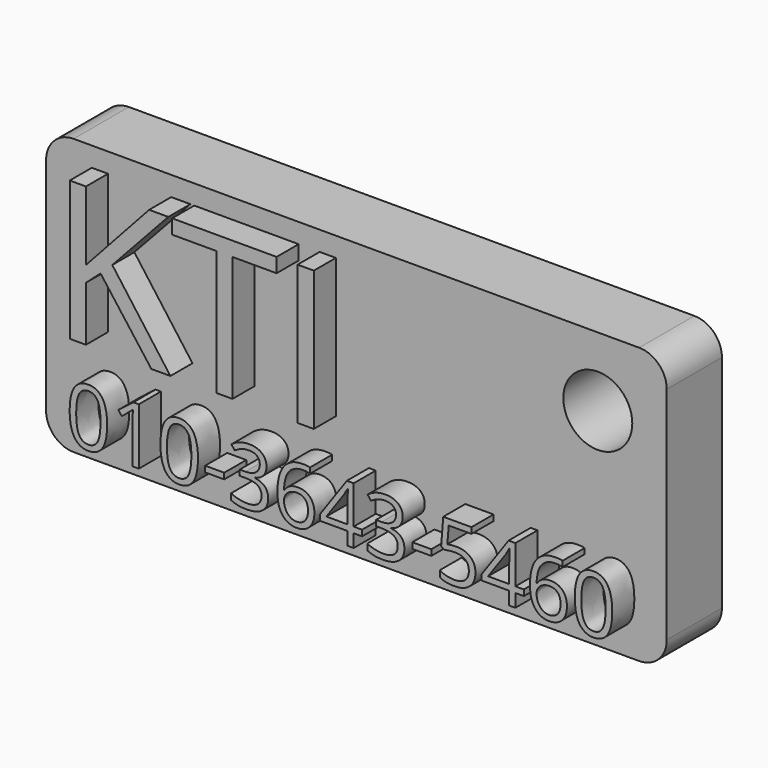
from build123d import *

# Parameters (mm, degrees)
F0_W         = 45
F0_H         = 20
F0_R         = 2.5
F1_DEPTH     = 5
F2_TEXT_SIZE = 14.1545947141
F3_DEPTH     = 2
F4_R         = 2
F5_TEXT_SIZE = 5.7574667146
F6_DEPTH     = 2


# Not quite as in the source:
# - Text() gives the source's letters only with a copy of the font that has no kerning and outlines rounded to 1/6400 em; it was checked with that copy


with BuildPart() as f1:
    # F0 (on Front) → F1 (new body)
    with BuildSketch(Plane.XZ):
        with Locations((22.5, 10)):
            Rectangle(F0_W, F0_H)
        with Locations((40, 15)):
            Circle(F0_R, mode=Mode.SUBTRACT)
    extrude(amount=F1_DEPTH)

    # F2 (on face) → F3 (join)
    with BuildSketch(Plane.XZ.offset(5)):
        with Locations((1.9274142686, 8.4753628975)):
            Text('KTI', F2_TEXT_SIZE, font='Open Sans', text_align=(TextAlign.LEFT, TextAlign.BOTTOM))
    extrude(amount=F3_DEPTH)

    # F4
    f4_edges = [f1.edges().sort_by_distance(p)[0] for p in [
        (45, -2.5, 20),
        (0, -2.5, 20),
        (45, -2.5, 0),
        (0, -2.5, 0),
    ]]
    fillet(f4_edges, radius=F4_R)

    # F5 (on face) → F6 (join)
    with BuildSketch(Plane.XZ.offset(5)):
        with Locations((3.0226701175, 1.8136018489)):
            Text('010-3643-5460', F5_TEXT_SIZE, font='Open Sans', text_align=(TextAlign.LEFT, TextAlign.BOTTOM))
    extrude(amount=F6_DEPTH)


solid = f1.part
